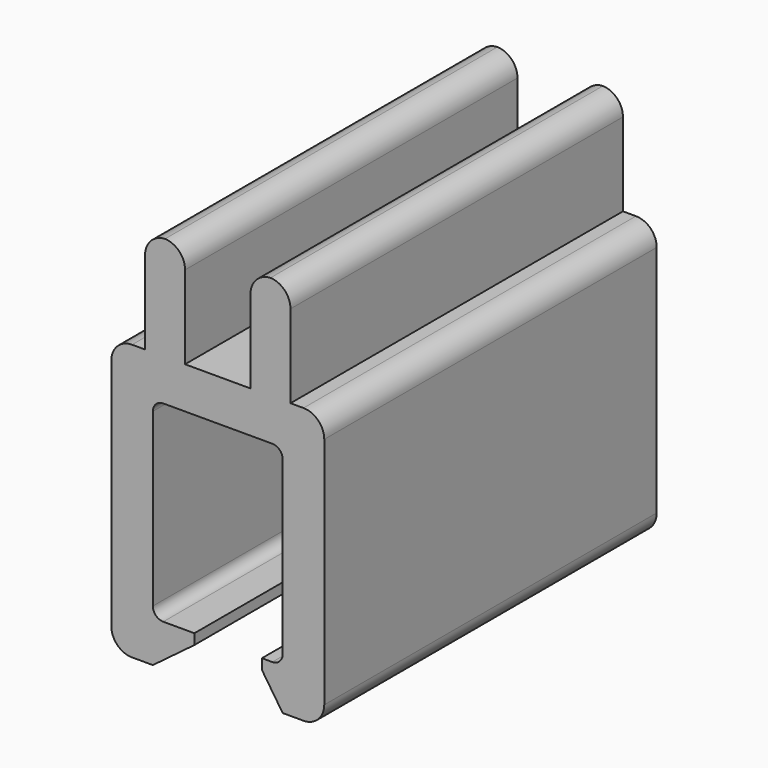
from build123d import *

# Parameters (mm, degrees)
F1_DEPTH     = 40
F2_R         = 2
F3_T1_DEPTH  = 50
F4_R         = 1
F5_TEXT_SIZE = 5.519552522
F6_DEPTH     = 0.4


# Not quite as in the source:
# - a fillet or chamfer that OpenCascade refuses, or shapes differently, is made with other operations: its cross-section is extruded or revolved along the edge and cut away or added
# - Text() gives the source's letters only with a copy of the font that has no kerning and outlines rounded to 1/6400 em; it was checked with that copy


with BuildPart() as f1:
    # F0 (on Front) → F1 (new body)
    with BuildSketch(Plane.XZ):
        Polygon((-16.5, 4), (-16.5, 22.5), (-4, 22.5), (-4, 4), (-6, 4), (-6, 3), (-4, 0), (0, 0), (0, 26.5), (-3.25, 26.5), (-3.25, 36.5), (-7.1, 36.5), (-7.1, 26.5), (-13.4, 26.5), (-13.4, 36.5), (-17.25, 36.5), (-17.25, 26.5), (-20.5, 26.5), (-20.5, 0), (-16.5, 0), (-12.5, 3), (-12.5, 4), align=None)
    extrude(amount=F1_DEPTH)

    # F2
    f2_edges = [f1.edges().sort_by_distance(p)[0] for p in [
        (0, -20, 26.5),
        (0, -20, 0),
        (-20.5, -20, 26.5),
        (-20.5, -20, 0),
    ]]
    fillet(f2_edges, radius=F2_R)

    # F3: fillet of radius 2 on 4 edges, made by hand

    # F3_s2 → F3_t1 (cut)
    with BuildSketch(Plane.XZ.offset(-5)):
        with BuildLine():
            ThreePointArc((-3.25, 34.5), (-3.8357864376, 35.9142135624), (-5.25, 36.5))
            Line((-5.25, 36.5), (-3.25, 36.5))
            Line((-3.25, 36.5), (-3.25, 34.5))
        make_face()
        with BuildLine():
            ThreePointArc((-15.25, 36.5), (-16.6642135624, 35.9142135624), (-17.25, 34.5))
            Line((-17.25, 34.5), (-17.25, 36.5))
            Line((-17.25, 36.5), (-15.25, 36.5))
        make_face()
        with BuildLine():
            ThreePointArc((-5.1, 36.5), (-6.5142135624, 35.9142135624), (-7.1, 34.5))
            Line((-7.1, 34.5), (-7.1, 36.5))
            Line((-7.1, 36.5), (-5.1, 36.5))
        make_face()
        with BuildLine():
            ThreePointArc((-13.4, 34.5), (-13.9857864376, 35.9142135624), (-15.4, 36.5))
            Line((-15.4, 36.5), (-13.4, 36.5))
            Line((-13.4, 36.5), (-13.4, 34.5))
        make_face()
    extrude(amount=F3_T1_DEPTH, mode=Mode.SUBTRACT)

    # F4
    f4_edges = [f1.edges().sort_by_distance(p)[0] for p in [
        (-16.5, -20, 22.5),
        (-4, -20, 22.5),
        (-16.5, -20, 4),
        (-4, -20, 4),
    ]]
    fillet(f4_edges, radius=F4_R)

    # F5 (on face) → F6 (cut)
    with BuildSketch(Plane(origin=(-20.5, 0, 0), x_dir=(0, -1, 0), z_dir=(-1, 0, 0))):
        with Locations((2.4220856523, 19.2355578042)):
            Text('Klipsofix', F5_TEXT_SIZE, font='Open Sans', text_align=(TextAlign.LEFT, TextAlign.BOTTOM))
        with Locations((2.4220856523, 11.7289663743)):
            Text('by', F5_TEXT_SIZE, font='Open Sans', text_align=(TextAlign.LEFT, TextAlign.BOTTOM))
        with Locations((2.4220856523, 4.2223749444)):
            Text('Benni & Chris', F5_TEXT_SIZE, font='Open Sans', text_align=(TextAlign.LEFT, TextAlign.BOTTOM))
    extrude(amount=-F6_DEPTH, mode=Mode.SUBTRACT)


solid = f1.part
